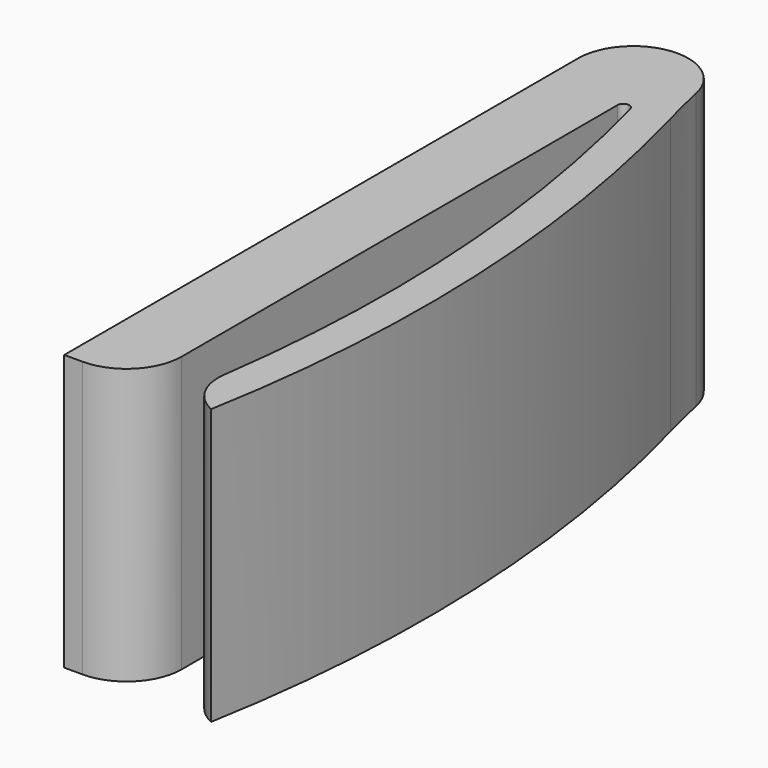
from build123d import *

# Parameters (mm, degrees)
F0_W        = 4
F0_H        = 35
F1_DEPTH    = 15
F2_T1_DEPTH = 15
F3_T1_DEPTH = 29.2746233567
F5_DEPTH    = 47
F6_DEPTH    = 5.1
F7_R        = 3
F8_R        = 43.7697785777


# Not quite as in the source:
# - a fillet or chamfer that OpenCascade refuses, or shapes differently, is made with other operations: its cross-section is extruded or revolved along the edge and cut away or added


with BuildPart() as f1:
    # F0 (on Top) → F1 (new body)
    with BuildSketch(Plane.XY):
        with Locations((-2, 17.5)):
            Rectangle(F0_W, F0_H)
        with BuildLine():
            Line((-4, 35), (0, 35))
            ThreePointArc((0, 35), (3.0631994803, 17.6178971132), (2, 0))
            Line((2, 0), (4, 0))
            ThreePointArc((4, 0), (5.0631994803, 17.6178971132), (2, 35))
            ThreePointArc((2, 35), (-1, 38), (-4, 35))
        make_face()
    extrude(amount=F1_DEPTH)

    # F2: fillet of radius 0.3232070394 on 1 edges, made by hand

    # F2_s2 → F2_t1 (join)
    with BuildSketch(Plane.XY):
        with BuildLine():
            ThreePointArc((0, 32.6758460939), (0.2811660755, 32.9963072424), (0.635477172, 32.7592136813))
            ThreePointArc((0.635477172, 32.7592136813), (0.3263947733, 33.8820616974), (0, 35))
            Line((0, 35), (0, 32.6758460939))
        make_face()
    extrude(amount=F2_T1_DEPTH)

    # F3: fillet of radius 2.6852748766 on 1 edges, made by hand

    # F3_s2 → F3_t1 (cut)
    with BuildSketch(Plane.XY.offset(-7.1373116784)):
        with BuildLine():
            ThreePointArc((2.4511484812, 2.8190530195), (2.7567902003, 1.1519659503), (4, 0))
            Line((4, 0), (2, 0))
            ThreePointArc((2, 0), (2.2389229437, 1.4073902438), (2.4511484812, 2.8190530195))
        make_face()
    extrude(amount=F3_T1_DEPTH, mode=Mode.SUBTRACT)

    # F4 (on face) → F5 (cut)
    with BuildSketch(Plane.XZ):
        with BuildLine():
            ThreePointArc((-3.15, 6.5), (-2, 5.35), (-0.85, 6.5))
            Line((-0.85, 6.5), (-2, 6.5))
            Line((-2, 6.5), (-3.15, 6.5))
        make_face()
        with BuildLine():
            ThreePointArc((-0.85, 6.5), (-1.0061251438, 7.0785436631), (-1.4321091654, 7.5))
            ThreePointArc((-1.4321091654, 7.5), (-2, 7.35), (-2.5678908346, 7.5))
            ThreePointArc((-2.5678908346, 7.5), (-2.9938748562, 7.0785436631), (-3.15, 6.5))
            Line((-3.15, 6.5), (-2, 6.5))
            Line((-2, 6.5), (-0.85, 6.5))
        make_face()
        with BuildLine():
            ThreePointArc((-2.5678908346, 7.5), (-2.9938748562, 7.9214563369), (-3.15, 8.5))
            Line((-3.15, 8.5), (-3.15, 6.5))
            ThreePointArc((-3.15, 6.5), (-2.9938748562, 7.0785436631), (-2.5678908346, 7.5))
        make_face()
        with BuildLine():
            Line((-0.85, 6.5), (-0.85, 8.5))
            ThreePointArc((-0.85, 8.5), (-1.0061251438, 7.9214563369), (-1.4321091654, 7.5))
            ThreePointArc((-1.4321091654, 7.5), (-1.0061251438, 7.0785436631), (-0.85, 6.5))
        make_face()
        with BuildLine():
            ThreePointArc((-1.4321091654, 7.5), (-1.0061251438, 7.9214563369), (-0.85, 8.5))
            Line((-0.85, 8.5), (-2, 8.5))
            Line((-2, 8.5), (-3.15, 8.5))
            ThreePointArc((-3.15, 8.5), (-2.9938748562, 7.9214563369), (-2.5678908346, 7.5))
            ThreePointArc((-2.5678908346, 7.5), (-2, 7.35), (-1.4321091654, 7.5))
        make_face()
        with BuildLine():
            Line((-2, 8.5), (-0.85, 8.5))
            ThreePointArc((-0.85, 8.5), (-2, 9.65), (-3.15, 8.5))
            Line((-3.15, 8.5), (-2, 8.5))
        make_face()
    extrude(amount=-F5_DEPTH, mode=Mode.SUBTRACT)

    # F4 (on face) → F6 (join)
    with BuildSketch(Plane.XZ):
        with BuildLine():
            Line((-2, 8.5), (-0.85, 8.5))
            ThreePointArc((-0.85, 8.5), (-2, 9.65), (-3.15, 8.5))
            Line((-3.15, 8.5), (-2, 8.5))
        make_face()
        with BuildLine():
            ThreePointArc((-1.4321091654, 7.5), (-1.0061251438, 7.9214563369), (-0.85, 8.5))
            Line((-0.85, 8.5), (-2, 8.5))
            Line((-2, 8.5), (-3.15, 8.5))
            ThreePointArc((-3.15, 8.5), (-2.9938748562, 7.9214563369), (-2.5678908346, 7.5))
            ThreePointArc((-2.5678908346, 7.5), (-2, 7.35), (-1.4321091654, 7.5))
        make_face()
        with BuildLine():
            ThreePointArc((-3.15, 6.5), (-2, 5.35), (-0.85, 6.5))
            Line((-0.85, 6.5), (-2, 6.5))
            Line((-2, 6.5), (-3.15, 6.5))
        make_face()
        with BuildLine():
            ThreePointArc((-0.85, 6.5), (-1.0061251438, 7.0785436631), (-1.4321091654, 7.5))
            ThreePointArc((-1.4321091654, 7.5), (-2, 7.35), (-2.5678908346, 7.5))
            ThreePointArc((-2.5678908346, 7.5), (-2.9938748562, 7.0785436631), (-3.15, 6.5))
            Line((-3.15, 6.5), (-2, 6.5))
            Line((-2, 6.5), (-0.85, 6.5))
        make_face()
        with BuildLine():
            Line((-0.85, 6.5), (-0.85, 8.5))
            ThreePointArc((-0.85, 8.5), (-1.0061251438, 7.9214563369), (-1.4321091654, 7.5))
            ThreePointArc((-1.4321091654, 7.5), (-1.0061251438, 7.0785436631), (-0.85, 6.5))
        make_face()
        with BuildLine():
            ThreePointArc((-2.5678908346, 7.5), (-2.9938748562, 7.9214563369), (-3.15, 8.5))
            Line((-3.15, 8.5), (-3.15, 6.5))
            ThreePointArc((-3.15, 6.5), (-2.9938748562, 7.0785436631), (-2.5678908346, 7.5))
        make_face()
    extrude(amount=-F6_DEPTH)

    # F7
    f7_edges = [f1.edges().sort_by_distance(p)[0] for p in [
        (0, 0, 7.5),
    ]]
    fillet(f7_edges, radius=F7_R)

    # F8
    f8_edges = [f1.edges().sort_by_distance(p)[0] for p in [
        (2, 35, 7.5),
    ]]
    fillet(f8_edges, radius=F8_R)


solid = f1.part
